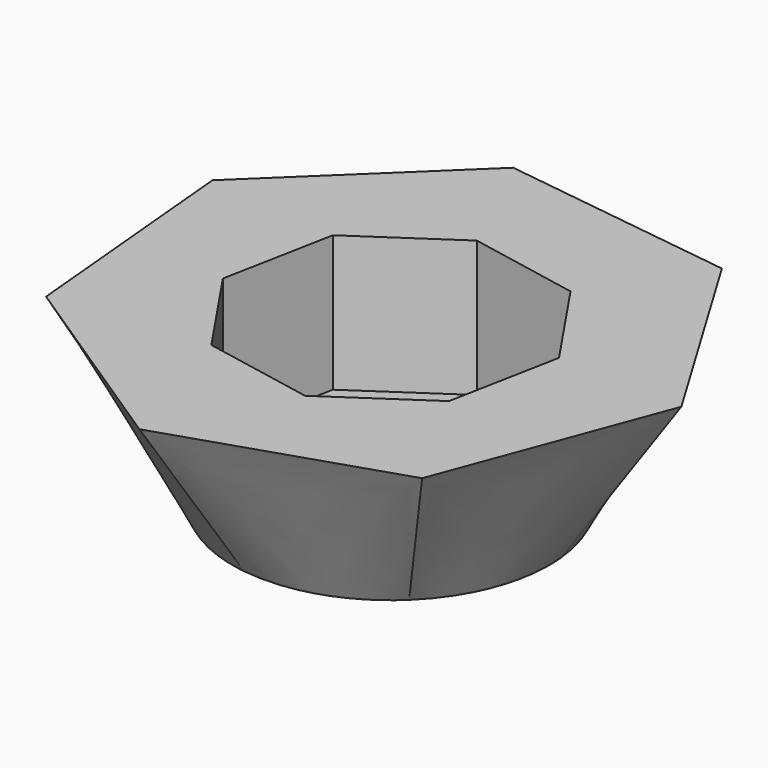
from build123d import *

# Parameters (mm, degrees)
F5_DEPTH = 25.4


# Not quite as in the source:
# - the arcs of a loft's sections are written as splines that run evenly, so that the points pair up as in the source's solid


with BuildPart() as f3:
    # F2 (on offset) → F3 section 0
    with BuildSketch(Plane.XY.offset(30.988)):
        Polygon((50.5604938488, 4.6280257192), (27.9056160827, 42.4153126988), (-15.7627597645, 48.2630041015), (-47.5614560073, 17.7676690299), (-43.5454057997, -26.1070832156), (-6.7387768606, -50.3226693123), (35.1422885006, -36.6442590214), align=None)
    # F0 (on Top) → F3 section 1
    with BuildSketch(Plane.XY):
        with BuildLine():
            add(Edge.make_bspline(
                [(29.4866381099, 2.699042457), (29.2174542384, 5.6398362877), (28.5051117676, 8.5396714595), (26.2570337959, 14.0012700055), (24.7215972806, 16.5623070077), (20.9635606735, 21.1186294397), (18.7414603862, 23.1133088958), (16.2744217872, 24.7364074332)],
                knots=[0, 0, 0, 0, 0.3333333333, 0.3333333333, 0.6666666667, 0.6666666667, 1, 1, 1, 1], degree=3))
            add(Edge.make_bspline(
                [(16.2744217872, 24.7364074332), (13.8073831882, 26.3595059706), (11.096062491, 27.6105918574), (5.424359114, 29.2582247193), (2.4647307492, 29.6545525654), (-3.440643072, 29.557221804), (-6.385603136, 29.0635761411), (-9.192766079, 28.1467530815)],
                knots=[0, 0, 0, 0, 0.3333333333, 0.3333333333, 0.6666666667, 0.6666666667, 1, 1, 1, 1], degree=3))
            add(Edge.make_bspline(
                [(-9.192766079, 28.1467530815), (-11.9999290219, 27.2299300218), (-14.6685481598, 25.8901734333), (-19.4929686175, 22.4831394605), (-21.6481283077, 20.4163151987), (-25.2539724079, 15.7386232925), (-26.7041772543, 13.1283777633), (-27.7376135895, 10.3620195702)],
                knots=[0, 0, 0, 0, 0.3333333333, 0.3333333333, 0.6666666667, 0.6666666667, 1, 1, 1, 1], degree=3))
            add(Edge.make_bspline(
                [(-27.7376135895, 10.3620195702), (-28.7710499246, 7.5956613772), (-29.3874428624, 4.6739263506), (-29.7316933959, -1.2222083845), (-29.4595052076, -4.1958239296), (-28.0505454335, -9.9314795677), (-26.9139612341, -12.6927568405), (-25.3954723229, -15.2255260241)],
                knots=[0, 0, 0, 0, 0.3333333333, 0.3333333333, 0.6666666667, 0.6666666667, 1, 1, 1, 1], degree=3))
            add(Edge.make_bspline(
                [(-25.3954723229, -15.2255260241), (-23.8769834116, -17.7582952077), (-21.976993695, -20.0618826048), (-17.5818466312, -24.0072083875), (-15.0872738217, -25.6484220597), (-9.7244856209, -28.1229757482), (-6.8569834599, -28.9559866583), (-3.9300224239, -29.3479399781)],
                knots=[0, 0, 0, 0, 0.3333333333, 0.3333333333, 0.6666666667, 0.6666666667, 1, 1, 1, 1], degree=3))
            add(Edge.make_bspline(
                [(-3.9300224239, -29.3479399781), (-1.003061388, -29.739893298), (1.9825799737, -29.690684771), (7.8074892511, -28.7142908169), (10.6459824762, -27.7872352464), (15.9243102077, -25.1372975861), (18.3634427166, -23.4147679279), (20.4948145181, -21.3707565397)],
                knots=[0, 0, 0, 0, 0.3333333333, 0.3333333333, 0.6666666667, 0.6666666667, 1, 1, 1, 1], degree=3))
            add(Edge.make_bspline(
                [(20.4948145181, -21.3707565397), (22.6261863196, -19.3267451516), (24.449230485, -16.961795725), (27.3176264836, -11.7989265964), (28.3625968311, -9.0016935363), (29.5817756531, -3.2227216343), (29.7558219815, -0.2417513736), (29.4866381099, 2.699042457)],
                knots=[0, 0, 0, 0, 0.3333333333, 0.3333333333, 0.6666666667, 0.6666666667, 1, 1, 1, 1], degree=3))
        make_face()
    loft(ruled=True)

    # F4 (on face) → F5 (cut)
    with BuildSketch(Plane.XY.offset(30.988)):
        Polygon((26.9755858675, 5.5309937743), (15.1636164888, 22.9856228979), (-5.5309937743, 26.9755858675), (-22.9856228979, 15.1636164888), (-26.9755858675, -5.5309937743), (-15.1636164888, -22.9856228979), (5.5309937743, -26.9755858675), (22.9856228979, -15.1636164888), align=None)
    extrude(amount=-F5_DEPTH, mode=Mode.SUBTRACT)


solid = f3.part
